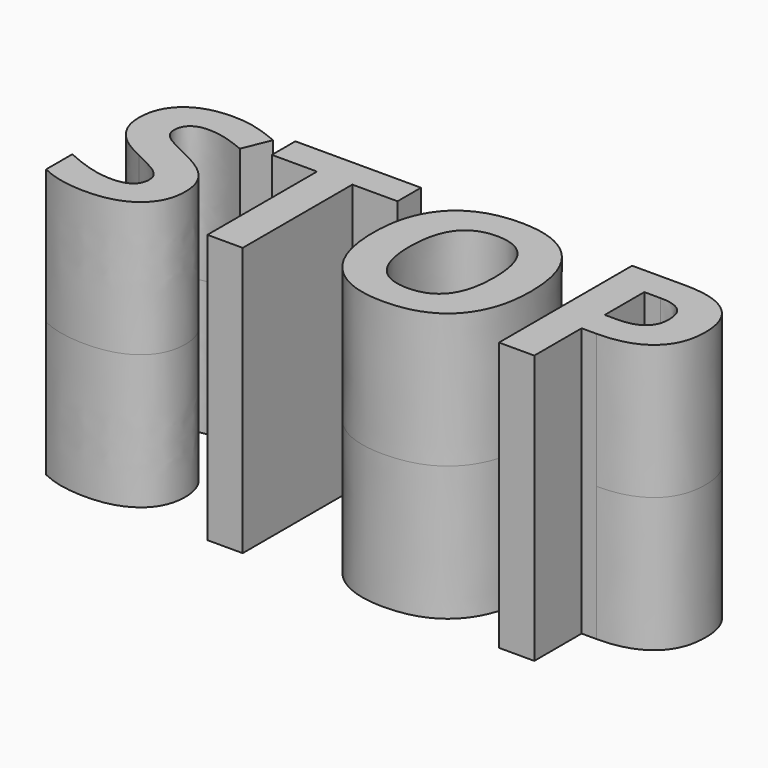
from build123d import *

# Parameters (mm, degrees)
F0_TEXT_SIZE = 22.0263506182
F1_DEPTH     = 12.7


# Not quite as in the source:
# - Text() gives the source's letters only with a copy of the font that has no kerning and outlines rounded to 1/6400 em; it was checked with that copy


with BuildPart() as f1:
    # F0 (on Top) → F1 (new body, symmetric)
    with BuildSketch(Plane.XY):
        with Locations((-27.9057334119, -8.153974959)):
            Text('STOP', F0_TEXT_SIZE, font='Open Sans', font_style=FontStyle.BOLD, text_align=(TextAlign.LEFT, TextAlign.BOTTOM))
    extrude(amount=F1_DEPTH, both=True)


solid = f1.part
